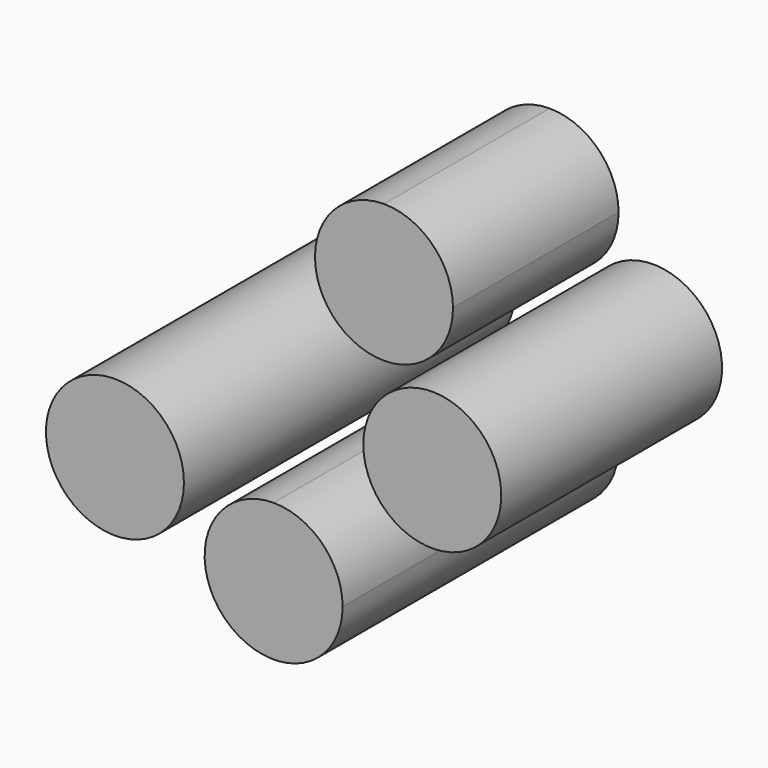
from build123d import *

# Parameters (mm, degrees)
F1_DEPTH = 76.2
F4_DEPTH = 127
F5_R     = 25.4
F6_DEPTH = 152.4
F7_DEPTH = 101.6


# Not quite as in the source:
# - the program builds the solid bodies; features that only make, move or delete a surface that nothing else refers to are left out


with BuildPart() as f1:
    # F0 (on Front) → F1 (new body)
    with BuildSketch(Plane.XZ):
        with BuildLine():
            ThreePointArc((25.4, 38.1), (17.9605122421, 56.0605122421), (0, 63.5))
            ThreePointArc((0, 63.5), (-25.4, 38.1), (0, 12.7))
            ThreePointArc((0, 12.7), (17.9605122421, 20.1394877579), (25.4, 38.1))
        make_face()
    extrude(amount=F1_DEPTH)


with BuildPart() as f4:
    # F3 (on Front) → F4 (new body)
    with BuildSketch(Plane.XZ):
        with BuildLine():
            ThreePointArc((0, -12.7), (-17.9605122421, -56.0605122421), (25.4, -38.1))
            ThreePointArc((25.4, -38.1), (17.9605122421, -20.1394877579), (0, -12.7))
        make_face()
    extrude(amount=F4_DEPTH)


with BuildPart() as f6:
    # F5 (on Front) → F6 (new body)
    with BuildSketch(Plane.XZ):
        with Locations((-38.1, 0)):
            Circle(F5_R)
    extrude(amount=F6_DEPTH)


with BuildPart() as f7:
    # F5 (on Front) → F7 (new body)
    with BuildSketch(Plane.XZ):
        with BuildLine():
            ThreePointArc((63.5, 0), (38.1, 25.4), (12.7, 0))
            ThreePointArc((12.7, 0), (38.1, -25.4), (63.5, 0))
        make_face()
    extrude(amount=F7_DEPTH)


solid = Compound([f1.part, f4.part, f6.part, f7.part])
